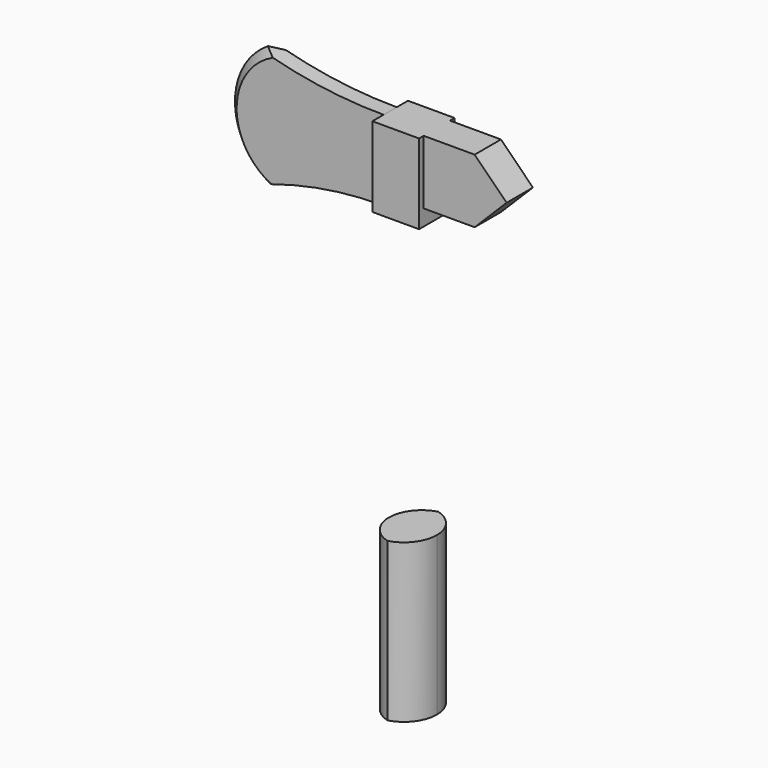
from build123d import *

# Parameters (mm, degrees)
F2_DEPTH    = 5.08
F3_T1_DEPTH = 49.8149751961
F5_DEPTH    = 3.429
F6_DEPTH    = 1.27
F7_T2_ANGLE = 164.598317353
F7_T4_ANGLE = 164.598317353
F1_W        = 12.957720086
F1_H        = 9.8736736098
F8_DEPTH    = 2.54
F9_T1_DEPTH = 31.2082991577


# Not quite as in the source:
# - a fillet or chamfer that OpenCascade refuses, or shapes differently, is made with other operations: its cross-section is extruded or revolved along the edge and cut away or added
# - the program builds the solid bodies; features that only make, move or delete a surface that nothing else refers to are left out


with BuildPart() as f2:
    # F0 (on Front) → F2 (new body, symmetric)
    with BuildSketch(Plane.XZ):
        Polygon((-3.9172582328, -39.270516485), (-7.3943706229, -39.270516485), (-7.3943706229, -63.6854916811), (0, -63.6854916811), (0, -39.270516485), align=None)
    extrude(amount=F2_DEPTH, both=True)

    # F3: fillet of radius 5.08 on 4 edges, made by hand

    # F3_s2 → F3_t1 (cut)
    with BuildSketch(Plane.XY.offset(-76.3854916811)):
        with BuildLine():
            ThreePointArc((-2.3143706229, -5.08), (-5.9064730714, -3.5921024484), (-7.3943706229, 0))
            Line((-7.3943706229, 0), (-7.3943706229, -5.08))
            Line((-7.3943706229, -5.08), (-2.3143706229, -5.08))
        make_face()
        with BuildLine():
            ThreePointArc((0, 0), (-1.4878975516, -3.5921024484), (-5.08, -5.08))
            Line((-5.08, -5.08), (0, -5.08))
            Line((0, -5.08), (0, 0))
        make_face()
        with BuildLine():
            ThreePointArc((-5.08, 5.08), (-1.4878975516, 3.5921024484), (0, 0))
            Line((0, 0), (0, 5.08))
            Line((0, 5.08), (-5.08, 5.08))
        make_face()
        with BuildLine():
            ThreePointArc((-2.3143706229, 5.08), (-5.9064730714, 3.5921024484), (-7.3943706229, 0))
            Line((-7.3943706229, 0), (-7.3943706229, 5.08))
            Line((-7.3943706229, 5.08), (-2.3143706229, 5.08))
        make_face()
    extrude(amount=F3_T1_DEPTH, mode=Mode.SUBTRACT)


with BuildPart() as f5:
    # F1 (on Front) → F5 (new body, symmetric)
    with BuildSketch(Plane.XZ):
        Polygon((-7.210094016, 16.0689561734), (-7.210094016, 3.7220644299), (0, 3.7220644299), (0, 6.1952825636), (0, 16.0689561734), align=None)
    extrude(amount=F5_DEPTH, both=True)

    # F1 (on Front) → F6 (join, symmetric)
    with BuildSketch(Plane.XZ):
        with BuildLine():
            ThreePointArc((-27.3404738286, 0), (-17.4458885018, 2.7837284893), (-7.210094016, 3.7220644299))
            Line((-7.210094016, 3.7220644299), (-7.210094016, 16.0689561734))
            ThreePointArc((-7.210094016, 16.0689561734), (-17.3911666381, 16.8392039186), (-27.3404738286, 19.1324129701))
            ThreePointArc((-27.3404738286, 19.1324129701), (-32.1990065296, 9.566206485), (-27.3404738286, 0))
        make_face()
    extrude(amount=F6_DEPTH, both=True)

    # F7: chamfer of 2.286 on 2 edges, made by hand

    # F7_s1 → F7_t2 (revolve, cut)
    with BuildSketch(Plane(origin=(-18.7162873139, 0, -2.5308211801), x_dir=(0, 1, 0), z_dir=(0.9909812322, 0, 0.1340007369))):
        Polygon((1.016, 24.0540768802), (-1.27, 21.7680768802), (-1.27, 24.0540768802), align=None)
    revolve(axis=Axis((-20.3520505033, -1.27, 9.566206485), (0, -1, 0)), revolution_arc=F7_T2_ANGLE, mode=Mode.SUBTRACT)

    # F7_s3 → F7_t4 (revolve, cut)
    with BuildSketch(Plane(origin=(-18.7162873139, 0, -2.5308211801), x_dir=(0, 1, 0), z_dir=(0.9909812322, 0, 0.1340007369))):
        Polygon((1.27, 21.7680768802), (-1.016, 24.0540768802), (1.27, 24.0540768802), align=None)
    revolve(axis=Axis((-20.3520505033, 1.27, 9.566206485), (0, -1, 0)), revolution_arc=F7_T4_ANGLE, mode=Mode.SUBTRACT)

    # F1 (on Front) → F8 (join, symmetric)
    with BuildSketch(Plane.XZ):
        with Locations((6.478860043, 11.1321193685)):
            Rectangle(F1_W, F1_H)
    extrude(amount=F8_DEPTH, both=True)

    # F9: chamfer of 5.08 on 2 edges, made by hand

    # F9_s2 → F9_t1 (cut)
    with BuildSketch(Plane.XZ.offset(-15.6041495789)):
        Polygon((7.877720086, 16.0689561734), (12.957720086, 10.9889561734), (12.957720086, 16.0689561734), align=None)
        Polygon((7.877720086, 6.1952825636), (12.957720086, 11.2752825636), (12.957720086, 6.1952825636), align=None)
    extrude(amount=F9_T1_DEPTH, mode=Mode.SUBTRACT)


solid = Compound([f2.part, f5.part])
